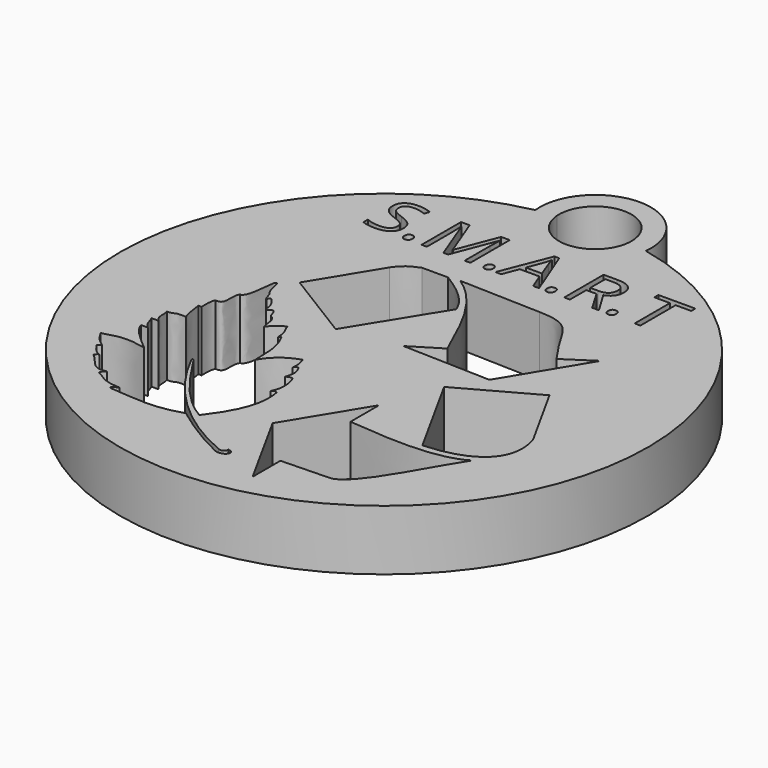
from build123d import *

# Parameters (mm, degrees)
F0_R         = 22.225
F1_DEPTH     = 5.08
F2_TEXT_SIZE = 5.8046777361
F3_DEPTH     = 25.4
F4_R         = 4.6831560321
F4_R_2       = 3.048
F5_DEPTH     = 5.08
F6_DEPTH     = 25.4


# Not quite as in the source:
# - Text() gives the source's letters only with a copy of the font that has no kerning and outlines rounded to 1/6400 em; it was checked with that copy


with BuildPart() as f1:
    # F0 (on Top) → F1 (new body)
    with BuildSketch(Plane.XY):
        Circle(F0_R)
        with BuildLine():
            add(Edge.make_bspline(
                [(-3.6698558833, -14.848462306), (-2.0807958208, -12.8078078851), (-1.3465294614, -10.9947733581), (-1.7013675533, -9.1921593994)],
                knots=[0, 0, 0, 0, 5.9890490795, 5.9890490795, 5.9890490795, 5.9890490795], degree=3))
            add(Edge.make_bspline(
                [(-8.83240439, -9.0056229383), (-7.4146692641, -11.2512307242), (-5.8154240251, -13.6142941192), (-3.6698558833, -14.848462306)],
                knots=[0, 0, 0, 0, 7.7968377539, 7.7968377539, 7.7968377539, 7.7968377539], degree=3))
            add(Edge.make_bspline(
                [(-9.0041141957, -9.0056229383), (-9.0344501659, -8.8549563661), (-8.9297788218, -8.8620521128), (-8.83240439, -9.0056229383)],
                knots=[0, 0, 0, 0, 0.1717098057, 0.1717098057, 0.1717098057, 0.1717098057], degree=3))
            add(Edge.make_bspline(
                [(0.3106326621, -17.7947264165), (-3.4093041904, -16.2692833692), (-6.8774651736, -13.2926767692), (-9.0041141957, -9.0056229383)],
                knots=[0, 0, 0, 0, 12.8067501333, 12.8067501333, 12.8067501333, 12.8067501333], degree=3))
            add(Edge.make_bspline(
                [(0.9027458145, -17.4735803157), (0.9027458145, -17.8147982806), (0.6217429182, -17.9653353989), (0.3106326621, -17.7947264165)],
                knots=[0, 0, 0, 0, 0.6735969145, 0.6735969145, 0.6735969145, 0.6735969145], degree=3))
            add(Edge.make_bspline(
                [(0.2102743601, -18.1058384478), (0.9930682136, -18.5474138707), (1.7858977662, -17.6542252302), (0.9027458145, -17.4735803157)],
                knots=[0, 0, 0, 0, 0.9376924127, 0.9376924127, 0.9376924127, 0.9376924127], degree=3))
            add(Edge.make_bspline(
                [(-4.5269043185, -15.1884481311), (-3.1115813181, -16.2692833692), (-1.3395877031, -17.377557233), (0.2102743601, -18.1058384478)],
                knots=[0, 0, 0, 0, 5.5634546905, 5.5634546905, 5.5634546905, 5.5634546905], degree=3))
            add(Edge.make_bspline(
                [(-10.6293894351, -15.4866958037), (-8.891412057, -15.5428359285), (-7.1385120973, -16.0610824823), (-4.5269043185, -15.1884481311)],
                knots=[0, 0, 0, 0, 6.1097689213, 6.1097689213, 6.1097689213, 6.1097689213], degree=3))
            add(Edge.make_bspline(
                [(-10.6642721221, -15.3116416186), (-10.7327736914, -15.3959607705), (-10.6905754656, -15.4592609033), (-10.6293894351, -15.4866958037)],
                knots=[0, 0, 0, 0, 0.1784958531, 0.1784958531, 0.1784958531, 0.1784958531], degree=3))
            add(Edge.make_bspline(
                [(-10.210079141, -15.0562040508), (-10.3614768013, -15.1413499067), (-10.5128744617, -15.2264957627), (-10.6642721221, -15.3116416186)],
                knots=[0, 0, 0, 0, 0.5210946317, 0.5210946317, 0.5210946317, 0.5210946317], degree=3))
            add(Edge.make_bspline(
                [(-12.6158809289, -14.2327323556), (-11.8352370337, -14.5876500756), (-11.7855602875, -14.9992676452), (-10.210079141, -15.0562040508)],
                knots=[0, 0, 0, 0, 2.5428306817, 2.5428306817, 2.5428306817, 2.5428306817], degree=3))
            add(Edge.make_bspline(
                [(-12.2852809727, -13.7715348974), (-12.3954809581, -13.9252673835), (-12.5520098954, -13.9772556722), (-12.6158809289, -14.2327323556)],
                knots=[0, 0, 0, 0, 0.567449933, 0.567449933, 0.567449933, 0.567449933], degree=3))
            add(Edge.make_bspline(
                [(-14.4786499441, -12.4762887135), (-13.7154590338, -13.0487717688), (-13.4896421805, -14.1076277941), (-12.2852809727, -13.7715348974)],
                knots=[0, 0, 0, 0, 2.5472593353, 2.5472593353, 2.5472593353, 2.5472593353], degree=3))
            add(Edge.make_bspline(
                [(-14.1794038936, -12.2080780566), (-14.3807958812, -12.2655360028), (-14.3789012606, -12.3868851612), (-14.4786499441, -12.4762887135)],
                knots=[0, 0, 0, 0, 0.4018521559, 0.4018521559, 0.4018521559, 0.4018521559], degree=3))
            add(Edge.make_bspline(
                [(-15.1921454817, -11.2669672817), (-14.9220814928, -11.6214547306), (-14.6098192781, -12.1109792963), (-14.1794038936, -12.2080780566)],
                knots=[0, 0, 0, 0, 1.3825104031, 1.3825104031, 1.3825104031, 1.3825104031], degree=3))
            add(Edge.make_bspline(
                [(-14.9474004284, -10.9969275072), (-14.9642787874, -11.148837395), (-15.1105637973, -11.1769540235), (-15.1921454817, -11.2669672817)],
                knots=[0, 0, 0, 0, 0.364447007, 0.364447007, 0.364447007, 0.364447007], degree=3))
            add(Edge.make_bspline(
                [(-16.0250011832, -9.7748385742), (-15.6900770962, -10.3638870642), (-15.4368914664, -10.6846150011), (-14.9474004284, -10.9969275072)],
                knots=[0, 0, 0, 0, 1.6293326078, 1.6293326078, 1.6293326078, 1.6293326078], degree=3))
            add(Edge.make_bspline(
                [(-12.4837169424, -9.6261715516), (-14.5914554596, -9.1220838949), (-15.0172607973, -9.5833297819), (-16.0250011832, -9.7748385742)],
                knots=[0, 0, 0, 0, 3.5444034699, 3.5444034699, 3.5444034699, 3.5444034699], degree=3))
            add(Edge.make_bspline(
                [(-14.6695198491, -7.2343968786), (-14.3146812916, -8.1924367696), (-13.3991986513, -8.8099502027), (-12.4837169424, -9.6261715516)],
                knots=[0, 0, 0, 0, 3.2401111761, 3.2401111761, 3.2401111761, 3.2401111761], degree=3))
            add(Edge.make_bspline(
                [(-14.094681479, -7.2343968786), (-14.2862942691, -7.2343968786), (-14.4779070591, -7.2343968786), (-14.6695198491, -7.2343968786)],
                knots=[0, 0, 0, 0, 0.5748383701, 0.5748383701, 0.5748383701, 0.5748383701], degree=3))
            add(Edge.make_bspline(
                [(-14.7475842386, -6.0365102254), (-14.5299499854, -6.4358057765), (-14.5914554596, -6.8227336742), (-14.094681479, -7.2343968786)],
                knots=[0, 0, 0, 0, 1.3642633351, 1.3642633351, 1.3642633351, 1.3642633351], degree=3))
            add(Edge.make_bspline(
                [(-14.1579201445, -6.0365102254), (-14.3544748425, -6.0365102254), (-14.5510295406, -6.0365102254), (-14.7475842386, -6.0365102254)],
                knots=[0, 0, 0, 0, 0.5896640942, 0.5896640942, 0.5896640942, 0.5896640942], degree=3))
            add(Edge.make_bspline(
                [(-14.5517848432, -4.6639125794), (-14.3787227571, -5.0518275239), (-14.6412989125, -5.5769523606), (-14.1579201445, -6.0365102254)],
                knots=[0, 0, 0, 0, 1.4279893902, 1.4279893902, 1.4279893902, 1.4279893902], degree=3))
            add(Edge.make_bspline(
                [(-13.0777778104, -4.4671325013), (-14.3608199432, -4.4132913463), (-13.6864762753, -4.6580340713), (-14.5517848432, -4.6639125794)],
                knots=[0, 0, 0, 0, 1.4870841038, 1.4870841038, 1.4870841038, 1.4870841038], degree=3))
            add(Edge.make_bspline(
                [(-13.4464818984, -2.7253171429), (-13.3045483381, -3.3690633718), (-13.3224502206, -4.1209841147), (-13.0777778104, -4.4671325013)],
                knots=[0, 0, 0, 0, 1.7804110332, 1.7804110332, 1.7804110332, 1.7804110332], degree=3))
            add(Edge.make_bspline(
                [(-13.1654646248, -2.7253171429), (-13.2591370493, -2.7253171429), (-13.3528094739, -2.7253171429), (-13.4464818984, -2.7253171429)],
                knots=[0, 0, 0, 0, 0.2810172737, 0.2810172737, 0.2810172737, 0.2810172737], degree=3))
            add(Edge.make_bspline(
                [(-13.0403060466, -1.4214821858), (-13.1905553862, -1.7066263827), (-13.2005913183, -2.1933875978), (-13.1654646248, -2.7253171429)],
                knots=[0, 0, 0, 0, 1.3098283342, 1.3098283342, 1.3098283342, 1.3098283342], degree=3))
            add(Edge.make_bspline(
                [(-12.2903939337, 0.2270568075), (-12.6854684204, -0.2221661562), (-12.0751466602, -1.6060974449), (-13.0403060466, -1.4214821858)],
                knots=[0, 0, 0, 0, 1.8110905526, 1.8110905526, 1.8110905526, 1.8110905526], degree=3))
            add(Edge.make_bspline(
                [(-11.4418696612, 3.0130427331), (-11.7840887979, 3.0978429131), (-11.5814739838, 0.2818405337), (-12.2903939337, 0.2270568075)],
                knots=[0, 0, 0, 0, 2.912337724, 2.912337724, 2.912337724, 2.912337724], degree=3))
            add(Edge.make_bspline(
                [(-10.8114546165, 1.4868918806), (-11.2807434052, 1.8732068129), (-11.2509047613, 3.0667316169), (-11.4418696612, 3.0130427331)],
                knots=[0, 0, 0, 0, 1.6512297093, 1.6512297093, 1.6512297093, 1.6512297093], degree=3))
            add(Edge.make_bspline(
                [(-10.5339586735, 0.7837613812), (-10.6879323721, 0.9037323762), (-10.7189559688, 1.2525150475), (-10.8114546165, 1.4868918806)],
                knots=[0, 0, 0, 0, 0.7559077309, 0.7559077309, 0.7559077309, 0.7559077309], degree=3))
            add(Edge.make_bspline(
                [(-10.2955959737, 1.0421724292), (-10.4131437838, 1.0078448104), (-10.4883890599, 0.9520701133), (-10.5339586735, 0.7837613812)],
                knots=[0, 0, 0, 0, 0.351558027, 0.351558027, 0.351558027, 0.351558027], degree=3))
            add(Edge.make_bspline(
                [(-9.8048551008, 0.3361352428), (-9.9267605692, 0.598026556), (-10.097200051, 0.8076647646), (-10.2955959737, 1.0421724292)],
                knots=[0, 0, 0, 0, 0.859834352, 0.859834352, 0.859834352, 0.859834352], degree=3))
            add(Edge.make_bspline(
                [(-9.5890099183, -0.418874668), (-9.7288200632, -0.3539445752), (-9.671873413, 0.1379038877), (-9.8048551008, 0.3361352428)],
                knots=[0, 0, 0, 0, 0.7852573516, 0.7852573516, 0.7852573516, 0.7852573516], degree=3))
            add(Edge.make_bspline(
                [(-9.0698245913, -0.272720994), (-9.1951452196, -0.1175494326), (-9.3861101195, -0.1682546863), (-9.5890099183, -0.418874668)],
                knots=[0, 0, 0, 0, 0.5393647191, 0.5393647191, 0.5393647191, 0.5393647191], degree=3))
            add(Edge.make_bspline(
                [(-8.6284577847, -0.9805023437), (-8.8697476313, -1.0514451424), (-8.9504718781, -0.3801508283), (-9.0698245913, -0.272720994)],
                knots=[0, 0, 0, 0, 0.834121752, 0.834121752, 0.834121752, 0.834121752], degree=3))
            add(Edge.make_bspline(
                [(-8.2121361047, -2.3495017085), (-8.4028262645, -1.6820656601), (-8.2671493292, -1.3468659017), (-8.6284577847, -0.9805023437)],
                knots=[0, 0, 0, 0, 1.4309028625, 1.4309028625, 1.4309028625, 1.4309028625], degree=3))
            add(Edge.make_bspline(
                [(-6.9826846011, -1.3409767998), (-7.4543925002, -1.6269637272), (-7.8207189217, -1.8928888021), (-8.2121361047, -2.3495017085)],
                knots=[0, 0, 0, 0, 1.5901803329, 1.5901803329, 1.5901803329, 1.5901803329], degree=3))
            add(Edge.make_bspline(
                [(-6.5611586906, -2.9618884437), (-6.6013038158, -1.8227602122), (-6.9927209988, -1.8678833731), (-6.9826846011, -1.3409767998)],
                knots=[0, 0, 0, 0, 1.6748249611, 1.6748249611, 1.6748249611, 1.6748249611], degree=3))
            add(Edge.make_bspline(
                [(-6.5611586906, -2.9618884437), (-6.4804106951, -2.8672087938), (-6.5025631338, -2.8165744152), (-6.3780373894, -2.8015153948)],
                knots=[0, 0, 0, 0, 0.2434192387, 0.2434192387, 0.2434192387, 0.2434192387], degree=3))
            add(Edge.make_bspline(
                [(-5.7114944793, -6.4368108287), (-5.7450733148, -4.3628914282), (-5.82102919, -3.8987100124), (-6.3780373894, -2.8015153948)],
                knots=[0, 0, 0, 0, 3.69589669, 3.69589669, 3.69589669, 3.69589669], degree=3))
            add(Edge.make_bspline(
                [(-3.2587943133, -4.4498392381), (-4.2792609893, -4.7421483323), (-5.2519864403, -5.4820356891), (-5.7114944793, -6.4368108287)],
                knots=[0, 0, 0, 0, 3.1565478306, 3.1565478306, 3.1565478306, 3.1565478306], degree=3))
            add(Edge.make_bspline(
                [(-3.1138474587, -5.7062930427), (-3.0051697977, -5.0884028897), (-3.2050856389, -4.7661298886), (-3.2587943133, -4.4498392381)],
                knots=[0, 0, 0, 0, 1.2647868413, 1.2647868413, 1.2647868413, 1.2647868413], degree=3))
            add(Edge.make_bspline(
                [(-2.7926845942, -5.4654544219), (-2.8980663046, -5.505588837), (-3.0034475494, -5.545723252), (-3.1138474587, -5.7062930427)],
                knots=[0, 0, 0, 0, 0.401433465, 0.401433465, 0.401433465, 0.401433465], degree=3))
            add(Edge.make_bspline(
                [(-2.6822849177, -7.0562250912), (-2.366140252, -6.1128418893), (-2.5869398378, -5.9070740826), (-2.7926845942, -5.4654544219)],
                knots=[0, 0, 0, 0, 1.5945969431, 1.5945969431, 1.5945969431, 1.5945969431], degree=3))
            add(Edge.make_bspline(
                [(-2.1485446487, -6.9422749802), (-2.2808315698, -6.8705943413), (-2.4815583602, -6.9207553752), (-2.6822849177, -7.0562250912)],
                knots=[0, 0, 0, 0, 0.545768543, 0.545768543, 0.545768543, 0.545768543], degree=3))
            add(Edge.make_bspline(
                [(-2.1485446487, -9.2285703868), (-1.7776532331, -8.5700359195), (-1.8060402945, -7.5693898834), (-2.1485446487, -6.9422749802)],
                knots=[0, 0, 0, 0, 2.2862954065, 2.2862954065, 2.2862954065, 2.2862954065], degree=3))
            add(Edge.make_bspline(
                [(-1.7013675533, -9.1921593994), (-1.8474544631, -8.9776925743), (-2.0858175121, -9.1482857242), (-2.1485446487, -9.2285703868)],
                knots=[0, 0, 0, 0, 0.4486570122, 0.4486570122, 0.4486570122, 0.4486570122], degree=3))
        make_face(mode=Mode.SUBTRACT)
        with BuildLine():
            Line((4.5568835922, -16.5921971202), (4.5568835922, -19.5228084922))
            Line((4.5568835922, -19.5228084922), (0.8138529956, -12.7362962812))
            Line((0.8138529956, -12.7362962812), (4.6831560321, -6.3712061383))
            Line((4.6831560321, -6.3712061383), (4.6831560321, -9.3789035454))
            add(Edge.make_bspline(
                [(4.6831560321, -9.3789035454), (7.7064465731, -9.6663367003), (12.1818231419, -10.0673492998), (14.3809635192, -8.6801880971)],
                knots=[0, 0, 0, 0, 9.7229457128, 9.7229457128, 9.7229457128, 9.7229457128], degree=3))
            add(Edge.make_bspline(
                [(14.3809635192, -8.6801880971), (12.6265883446, -11.3139841706), (10.2695953101, -16.5320113301), (8.5249813274, -16.4785459638)],
                knots=[0, 0, 0, 0, 9.752277316, 9.752277316, 9.752277316, 9.752277316], degree=3))
            Line((8.5249813274, -16.4785459638), (4.5568835922, -16.5921971202))
        make_face(mode=Mode.SUBTRACT)
        with BuildLine():
            add(Edge.make_bspline(
                [(10.4782309613, -9.0591871357), (14.2679118398, -8.8521425746), (16.6626591235, -7.2243604809), (15.660093934, -3.8947357042)],
                knots=[0, 0, 0, 0, 7.3159594351, 7.3159594351, 7.3159594351, 7.3159594351], degree=3))
            Line((10.4782309613, -9.0591871357), (6.3935037001, -1.6657470205))
            Line((6.3935037001, -1.6657470205), (12.5436153563, 1.7320662234))
            Line((12.5436153563, 1.7320662234), (15.660093934, -3.8947357042))
        make_face(mode=Mode.SUBTRACT)
        with BuildLine():
            Line((-4.3122945353, 0.306259346), (-10.3043522686, 4.0033864789))
            Line((-10.3043522686, 4.0033864789), (-7.0298193023, 9.3874614686))
            add(Edge.make_bspline(
                [(-5.3419158794, 10.6698684394), (-5.9326817282, 10.4169696569), (-6.4390525222, 10.2482317016), (-7.0298193023, 9.3874614686)],
                knots=[0, 0, 0, 0, 2.1198079167, 2.1198079167, 2.1198079167, 2.1198079167], degree=3))
            Line((-5.3419158794, 10.6698684394), (-3.147640964, 10.6698684394))
            add(Edge.make_bspline(
                [(0.1172371913, 7.485349727), (-0.446994818, 8.8466536254), (-1.7973177601, 9.8426556215), (-3.147640964, 10.6698684394)],
                knots=[0, 0, 0, 0, 4.5607662513, 4.5607662513, 4.5607662513, 4.5607662513], degree=3))
            Line((0.1172371913, 7.485349727), (-4.3122945353, 0.306259346))
        make_face(mode=Mode.SUBTRACT)
        with BuildLine():
            Line((0.66970638, 1.2064311886), (3.1449929811, 2.7289381251))
            add(Edge.make_bspline(
                [(3.1449929811, 2.7289381251), (1.7175605753, 5.8656730689), (0.5394982873, 8.9315958321), (-2.199851675, 10.7912290841)],
                knots=[0, 0, 0, 0, 9.6730501863, 9.6730501863, 9.6730501863, 9.6730501863], degree=3))
            Line((-2.199851675, 10.7912290841), (4.6147354878, 10.5758169666))
            add(Edge.make_bspline(
                [(9.6747480262, 6.0551590672), (7.23502459, 9.3870991841), (7.7698999085, 10.4951374233), (4.6147354878, 10.5758169666)],
                knots=[0, 0, 0, 0, 6.7852836883, 6.7852836883, 6.7852836883, 6.7852836883], degree=3))
            Line((9.6747480262, 6.0551590672), (12.1072186157, 7.6529849321))
            Line((12.1072186157, 7.6529849321), (8.0865584314, 0.9848668706))
            Line((8.0865584314, 0.9848668706), (0.66970638, 1.2064311886))
        make_face(mode=Mode.SUBTRACT)
    extrude(amount=F1_DEPTH)

    # F2 (on face) → F3 (cut)
    with BuildSketch(Plane.XY.offset(5.08)):
        with Locations((-12.7, 13.208)):
            Text('S.M.A.R.T', F2_TEXT_SIZE, font='Open Sans', text_align=(TextAlign.LEFT, TextAlign.BOTTOM))
    extrude(amount=-F3_DEPTH, mode=Mode.SUBTRACT)

    # F4 (on face) → F5 (join)
    with BuildSketch(Plane.XY.offset(5.08)):
        with Locations((0, 22.225)):
            Circle(F4_R)
        with Locations((0, 22.225)):
            Circle(F4_R_2, mode=Mode.SUBTRACT)
    extrude(amount=-F5_DEPTH)

    # F4 (on face) → F6 (cut)
    with BuildSketch(Plane.XY.offset(5.08)):
        with BuildLine():
            ThreePointArc((3.0408256463, 22.0159942857), (0, 22.225), (-3.0408256463, 22.0159942857))
            ThreePointArc((-3.0408256463, 22.0159942857), (0, 19.177), (3.0408256463, 22.0159942857))
        make_face()
    extrude(amount=-F6_DEPTH, mode=Mode.SUBTRACT)


solid = f1.part
